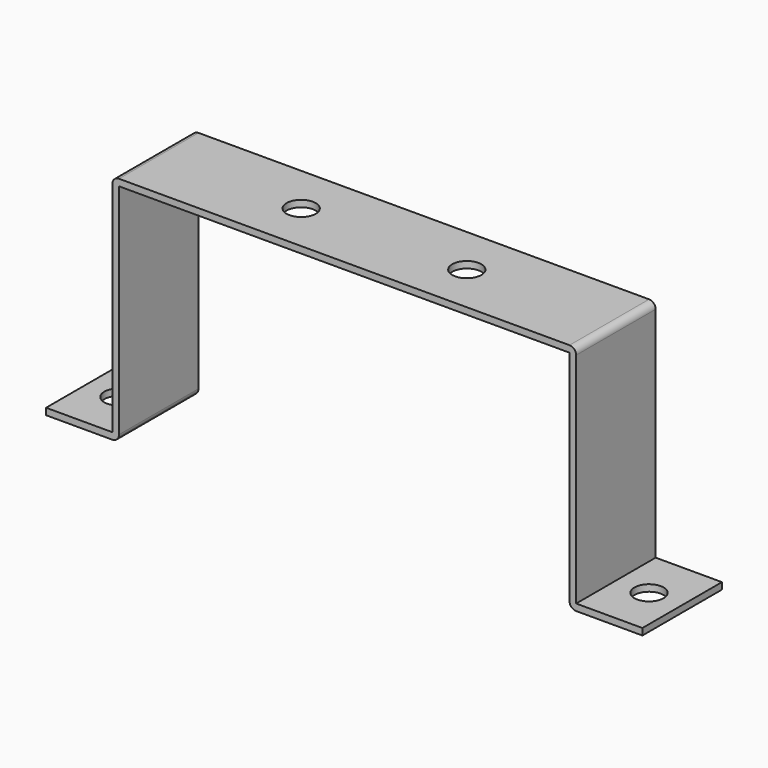
from build123d import *

# Parameters (mm, degrees)
F1_DEPTH = 30
F2_R     = 4.4
F3_R     = 4.4
F4_DEPTH = 25
F5_R     = 2
F6_R     = 2


# Not quite as in the source:
# - a feature names something its author has since deleted; it is built from what else it names


with BuildPart() as f1:
    # F0 (on Front) → F1 (new body)
    with BuildSketch(Plane.XZ):
        Polygon((90, -1), (90, 1), (70, 1), (70, 69), (-70, 69), (-70, 1), (-90, 1), (-90, -1), (-68, -1), (-68, 67), (68, 67), (68, -1), align=None)
    extrude(amount=F1_DEPTH)

    # F2 (on face) + F3 (on face) → F4 (cut)
    with BuildSketch(Plane.XY.offset(1)):
        with Locations((-80, -15)):
            Circle(F2_R)
        with Locations((80, -15)):
            Circle(F2_R)
    with BuildSketch(Plane.XY.offset(69)):
        with Locations((-25, -15)):
            Circle(F3_R)
        with Locations((25, -15)):
            Circle(F3_R)
    extrude(amount=-F4_DEPTH, mode=Mode.SUBTRACT)

    # F5
    f5_edges = [f1.edges().sort_by_distance(p)[0] for p in [
        (-70, -15, 69),
        (70, -15, 69),
    ]]
    fillet(f5_edges, radius=F5_R)

    # F6
    f6_edges = [f1.edges().sort_by_distance(p)[0] for p in [
        (68, -15, -1),
        (-68, -15, -1),
    ]]
    fillet(f6_edges, radius=F6_R)


solid = f1.part
